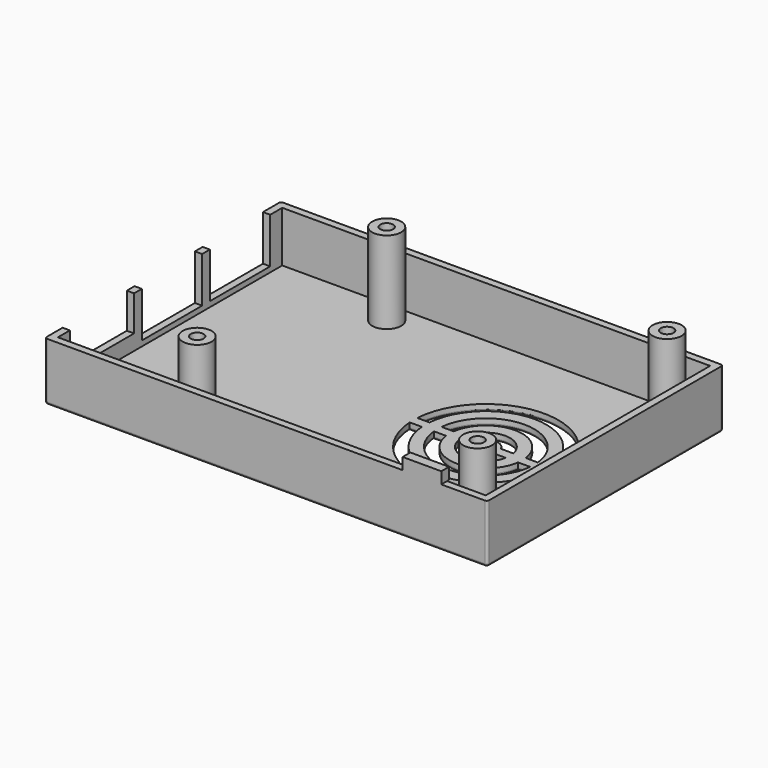
from build123d import *

# Parameters (mm, degrees)
F0_W      = 91.5
F0_H      = 61
F1_DEPTH  = 12
F2_T      = -1.5
F3_W      = 8
F3_H      = 2.4
F4_DEPTH  = 2
F5_W      = 16.6
F5_H      = 7.3
F5_W_2    = 15.6
F5_H_2    = 9.4
F6_DEPTH  = 2.1
F8_DEPTH  = 3
F9_R      = 1.25
F10_DEPTH = 3
F11_R     = 3
F11_R_2   = 1.325
F12_DEPTH = 17.05
F13_DEPTH = 25
F14_R     = 0.5
F15_R     = 0.5


with BuildPart() as f1:
    # F0 (on Top) → F1 (new body)
    with BuildSketch(Plane.XY):
        Rectangle(F0_W, F0_H)
    extrude(amount=F1_DEPTH)

    # F2
    f2_openings = [f1.faces().sort_by_distance(p)[0] for p in [
        (0, 0, 12),
    ]]
    offset(amount=F2_T, openings=f2_openings)

    # F3 (on face) → F4 (join)
    with BuildSketch(Plane.XZ.offset(30.5)):
        with Locations((32.25, 13.2)):
            Rectangle(F3_W, F3_H)
    extrude(amount=-F4_DEPTH)

    # F5 (on face) → F6 (cut)
    with BuildSketch(Plane(origin=(-45.75, 0, 0), x_dir=(0, -1, 0), z_dir=(-1, 0, 0))):
        with Locations((17.6, 8.35)):
            Rectangle(F5_W, F5_H)
        with Locations((-0.5, 7.3)):
            Rectangle(F5_W_2, F5_H_2)
        with Locations((-18.1, 7.3)):
            Rectangle(F5_W_2, F5_H_2)
    extrude(amount=-F6_DEPTH, mode=Mode.SUBTRACT)

    # F7 (on face) → F8 (cut)
    with BuildSketch(Plane(origin=(0, 0, 0), x_dir=(1, 0, 0), z_dir=(0, 0, -1))):
        with BuildLine():
            ThreePointArc((18.7729597218, 0.9874563896), (21.0696812719, 2.5), (23.366402822, 0.9874563896))
            Line((23.366402822, 0.9874563896), (25.9712044922, 0.9874563896))
            ThreePointArc((25.9712044922, 0.9874563896), (21.0696812719, 5), (16.1681580517, 0.9874563896))
            Line((16.1681580517, 0.9874563896), (18.7729597218, 0.9874563896))
        make_face()
        with BuildLine():
            Line((25.9712044922, -0.9874563896), (23.366402822, -0.9874563896))
            ThreePointArc((23.366402822, -0.9874563896), (21.0696812719, -2.5), (18.7729597218, -0.9874563896))
            Line((18.7729597218, -0.9874563896), (16.1681580517, -0.9874563896))
            ThreePointArc((16.1681580517, -0.9874563896), (21.0696812719, -5), (25.9712044922, -0.9874563896))
        make_face()
        with BuildLine():
            ThreePointArc((13.6349701223, 0.9874563896), (21.0696812719, 7.5), (28.5043924216, 0.9874563896))
            Line((28.5043924216, 0.9874563896), (31.0208083377, 0.9874563896))
            ThreePointArc((31.0208083377, 0.9874563896), (21.0696812719, 10), (11.1185542062, 0.9874563896))
            Line((11.1185542062, 0.9874563896), (13.6349701223, 0.9874563896))
        make_face()
        with BuildLine():
            Line((31.0208083377, -0.9874563896), (28.5043924216, -0.9874563896))
            ThreePointArc((28.5043924216, -0.9874563896), (21.0696812719, -7.5), (13.6349701223, -0.9874563896))
            Line((13.6349701223, -0.9874563896), (11.1185542062, -0.9874563896))
            ThreePointArc((11.1185542062, -0.9874563896), (21.0696812719, -10), (31.0208083377, -0.9874563896))
        make_face()
        with BuildLine():
            ThreePointArc((8.6087451161, 0.9874563896), (21.0696812719, 12.5), (33.5306174277, 0.9874563896))
            Line((33.5306174277, 0.9874563896), (36.0371436446, 0.9874563896))
            ThreePointArc((36.0371436446, 0.9874563896), (21.0696812719, 15), (6.1022188992, 0.9874563896))
            Line((6.1022188992, 0.9874563896), (8.6087451161, 0.9874563896))
        make_face()
        with BuildLine():
            Line((36.0371436446, -0.9874563896), (33.5306174277, -0.9874563896))
            ThreePointArc((33.5306174277, -0.9874563896), (21.0696812719, -12.5), (8.6087451161, -0.9874563896))
            Line((8.6087451161, -0.9874563896), (6.1022188992, -0.9874563896))
            ThreePointArc((6.1022188992, -0.9874563896), (21.0696812719, -15), (36.0371436446, -0.9874563896))
        make_face()
    extrude(amount=-F8_DEPTH, mode=Mode.SUBTRACT)

    # F9 (on face) → F10 (cut)
    with BuildSketch(Plane(origin=(0, 0, 0), x_dir=(1, 0, 0), z_dir=(0, 0, -1))):
        with Locations((21.0696812719, 0)):
            Circle(F9_R)
    extrude(amount=-F10_DEPTH, mode=Mode.SUBTRACT)

    # F11 (on face) → F12 (join)
    with BuildSketch(Plane.XY.offset(1.5)):
        with Locations((38.96, 24.5)):
            Circle(F11_R)
        with Locations((38.96, 24.5)):
            Circle(F11_R_2, mode=Mode.SUBTRACT)
        with Locations((38.96, -24.5)):
            Circle(F11_R)
        with Locations((38.96, -24.5)):
            Circle(F11_R_2, mode=Mode.SUBTRACT)
        with Locations((-19.04, 24.5)):
            Circle(F11_R)
        with Locations((-19.04, 24.5)):
            Circle(F11_R_2, mode=Mode.SUBTRACT)
        with Locations((-19.04, -24.5)):
            Circle(F11_R)
        with Locations((-19.04, -24.5)):
            Circle(F11_R_2, mode=Mode.SUBTRACT)
    extrude(amount=F12_DEPTH)

    # F13 (cut): faces of the model
    f13_faces = [f1.faces().sort_by_distance(p)[0] for p in [
        (38.96, 24.5, 1.5),
        (38.96, -24.5, 1.5),
        (-19.04, -24.5, 1.5),
        (-19.04, 24.5, 1.5),
    ]]
    extrude(f13_faces, amount=-F13_DEPTH, mode=Mode.SUBTRACT)

    # F14
    f14_edges = [f1.edges().sort_by_distance(p)[0] for p in [
        (0, 30.5, 0),
        (45.75, 0, 0),
        (0, -30.5, 0),
        (-45.75, 0, 0),
        (45.75, -30.5, 6),
        (-45.75, -30.5, 6),
        (-45.75, 30.5, 6),
        (45.75, 30.5, 6),
    ]]
    fillet(f14_edges, radius=F14_R)

    # F15
    f15_edges = [f1.edges().sort_by_distance(p)[0] for p in [
        (21.069681, 15, 0),
        (21.069681, -15, 0),
        (34.783881, 0.987456, 0),
        (34.783881, -0.987456, 0),
        (21.069681, 12.5, 0),
        (21.069681, -12.5, 0),
        (7.355482, -0.987456, 0),
        (7.355482, 0.987456, 0),
        (21.069681, -10, 0),
        (21.069681, 10, 0),
        (21.069681, 7.5, 0),
        (21.069681, -7.5, 0),
        (12.376762, -0.987456, 0),
        (29.7626, 0.987456, 0),
        (21.069681, 5, 0),
        (17.470559, 0.987456, 0),
        (21.069681, -5, 0),
        (24.668804, -0.987456, 0),
        (17.470559, -0.987456, 0),
        (24.668804, 0.987456, 0),
        (12.376762, 0.987456, 0),
        (29.7626, -0.987456, 0),
        (21.069681, 2.5, 0),
        (21.069681, -2.5, 0),
        (19.819681, 0, 0),
    ]]
    fillet(f15_edges, radius=F15_R)


solid = f1.part
